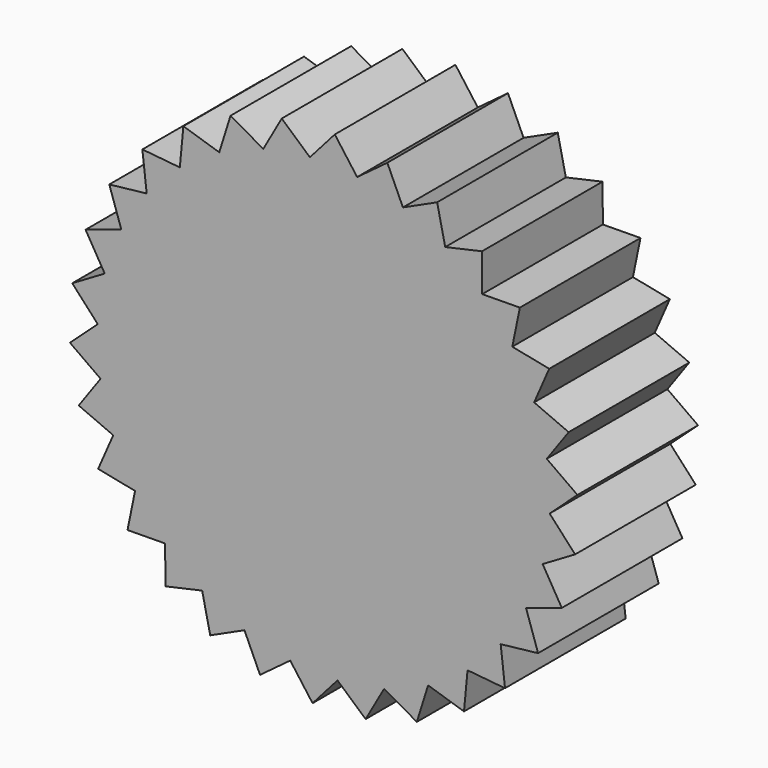
from build123d import *

# Parameters (mm, degrees)
F0_R            = 38.1
F1_DEPTH        = 25.4
F3_DEPTH        = 25.4
F3_COPIES_COUNT = 30


# Not quite as in the source:
# - a pattern or mirror of a feature is missing from the dataset's text; its kind, count and spacing are read off the source's solid


with BuildPart() as f1:
    # F0 (on Front) → F1 (new body)
    with BuildSketch(Plane.XZ):
        Circle(F0_R)
    extrude(amount=F1_DEPTH)

    # F2 (on face) → F3 (join)
    with BuildSketch(Plane.XZ.offset(25.4)):
        with BuildLine():
            Line((1.8707504496, 42.7830666304), (-2.323463975, 38.0290877508))
            ThreePointArc((-2.323463975, 38.0290877508), (1.6643863058, 38.0636285478), (5.6340012219, 37.6811362651))
            Line((5.6340012219, 37.6811362651), (1.8707504496, 42.7830666304))
        make_face()
    f3 = extrude(amount=-F3_DEPTH)

    # F3_copies: F3 ×30 about axis
    f3_copies_axis = Axis((0, 0, 0), (0, 1, 0))
    for i in range(1, F3_COPIES_COUNT):
        add(f3.rotate(f3_copies_axis, i * 360 / F3_COPIES_COUNT))


solid = f1.part
